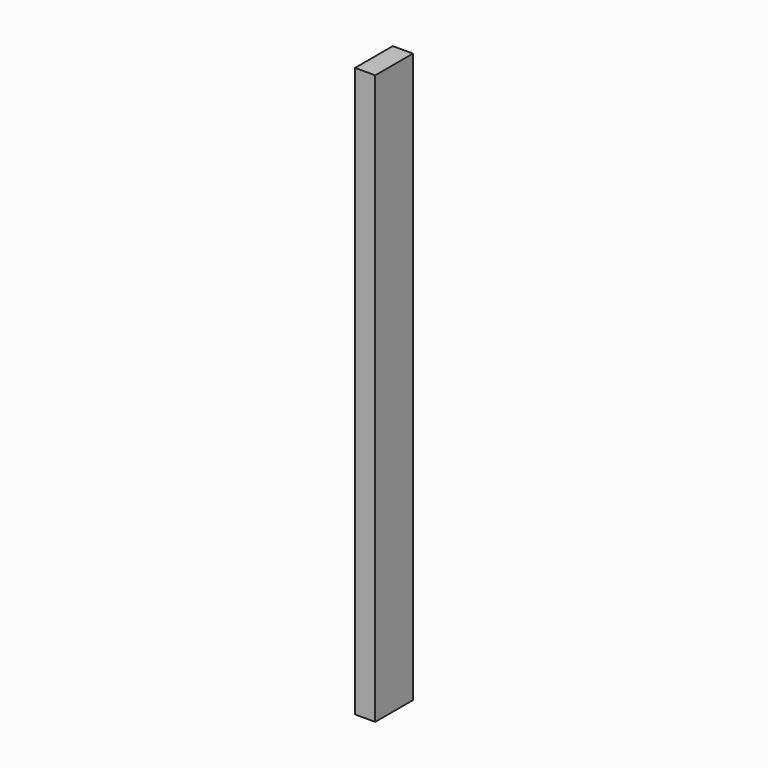
from build123d import *

# Parameters (mm, degrees)
F0_W     = 38.1
F0_H     = 88.9
F1_DEPTH = 1073.15


# Not quite as in the source:
# - a feature names something its author has since deleted; it is built from what else it names


with BuildPart() as f1:
    # F0 (on Top) → F1 (new body)
    with BuildSketch(Plane.XY):
        Rectangle(F0_W, F0_H)
    extrude(amount=F1_DEPTH)


solid = f1.part
